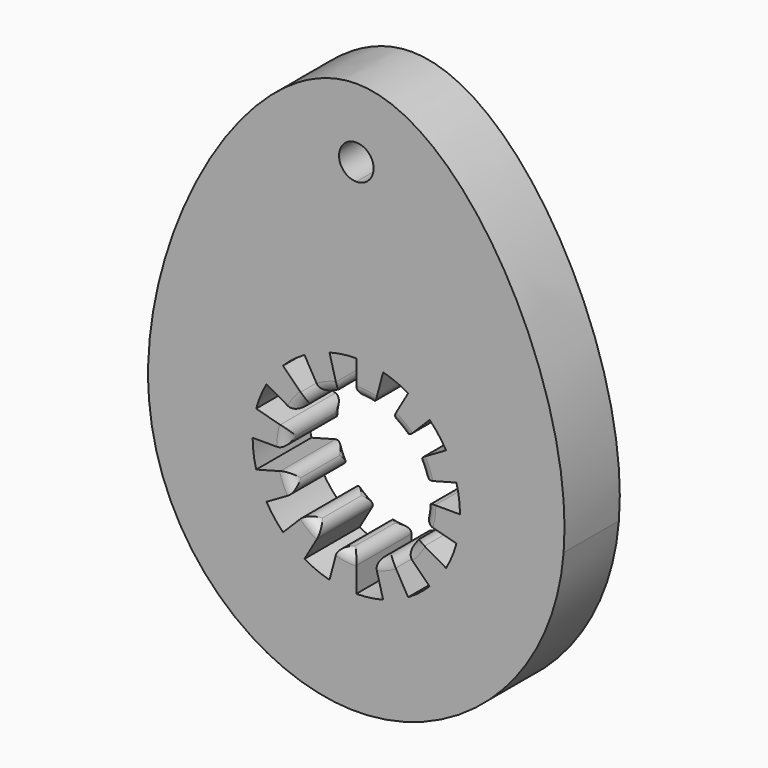
from build123d import *

# Parameters (mm, degrees)
F1_DEPTH = 12.7
F2_R     = 1.905


with BuildPart() as f1:
    # F0 (on Front) → F1 (new body)
    with BuildSketch(Plane.XZ):
        with BuildLine():
            ThreePointArc((18.4008869908, 4.9305028092), (18.8870246092, 2.4865239618), (19.05, 0))
            Line((19.05, 0), (38.1, 0))
            add(Edge.make_bspline(
                [(38.1, 0), (40.2886501107, 26.66795404), (20.1443250553, 63.5), (0, 63.5)],
                knots=[0.7301671149, 0.7301671149, 0.7301671149, 0.7301671149, 1, 1, 1, 1], degree=3))
            Line((0, 63.5), (0, 53.975))
            ThreePointArc((0, 53.975), (2.2450640303, 53.0450640303), (3.175, 50.8))
            ThreePointArc((3.175, 50.8), (2.2450640303, 48.5549359697), (0, 47.625))
            Line((0, 47.625), (0, 19.05))
            ThreePointArc((0, 19.05), (2.4865239618, 18.8870246092), (4.9305028092, 18.4008869908))
            ThreePointArc((4.9305028092, 18.4008869908), (7.2901193866, 17.5999050943), (9.525, 16.4977839421))
            ThreePointArc((9.525, 16.4977839421), (11.5969052226, 15.1133811325), (13.4703841816, 13.4703841816))
            ThreePointArc((13.4703841816, 13.4703841816), (15.1133811325, 11.5969052226), (16.4977839421, 9.525))
            ThreePointArc((16.4977839421, 9.525), (17.5999050943, 7.2901193866), (18.4008869908, 4.9305028092))
        make_face()
        with BuildLine():
            Line((38.1, 0), (19.05, 0))
            ThreePointArc((19.05, 0), (18.8870246092, -2.4865239618), (18.4008869908, -4.9305028092))
            ThreePointArc((18.4008869908, -4.9305028092), (17.5999050943, -7.2901193866), (16.4977839421, -9.525))
            ThreePointArc((16.4977839421, -9.525), (15.1133811325, -11.5969052226), (13.4703841816, -13.4703841816))
            ThreePointArc((13.4703841816, -13.4703841816), (11.5969052226, -15.1133811325), (9.525, -16.4977839421))
            ThreePointArc((9.525, -16.4977839421), (7.2901193866, -17.5999050943), (4.9305028092, -18.4008869908))
            ThreePointArc((4.9305028092, -18.4008869908), (2.4865239618, -18.8870246092), (0, -19.05))
            Line((0, -19.05), (0, -38.1))
            add(Edge.make_bspline(
                [(0, -38.1), (18.1165420908, -38.1), (36.2330841816, -22.7477315801), (38.1, 0)],
                knots=[0.5, 0.5, 0.5, 0.5, 0.7301671149, 0.7301671149, 0.7301671149, 0.7301671149], degree=3))
        make_face()
        with BuildLine():
            ThreePointArc((-18.4008869908, -4.9305028092), (-18.8870246092, -2.4865239618), (-19.05, 0))
            Line((-19.05, 0), (-38.1, 0))
            add(Edge.make_bspline(
                [(-38.1, 0), (-36.2330841816, -22.7477315801), (-18.1165420908, -38.1), (0, -38.1)],
                knots=[0.2698328851, 0.2698328851, 0.2698328851, 0.2698328851, 0.5, 0.5, 0.5, 0.5], degree=3))
            Line((0, -38.1), (0, -19.05))
            ThreePointArc((0, -19.05), (-2.4865239618, -18.8870246092), (-4.9305028092, -18.4008869908))
            ThreePointArc((-4.9305028092, -18.4008869908), (-7.2901193866, -17.5999050943), (-9.525, -16.4977839421))
            ThreePointArc((-9.525, -16.4977839421), (-11.5969052226, -15.1133811325), (-13.4703841816, -13.4703841816))
            ThreePointArc((-13.4703841816, -13.4703841816), (-15.1133811325, -11.5969052226), (-16.4977839421, -9.525))
            ThreePointArc((-16.4977839421, -9.525), (-17.5999050943, -7.2901193866), (-18.4008869908, -4.9305028092))
        make_face()
        with BuildLine():
            Line((-38.1, 0), (-19.05, 0))
            ThreePointArc((-19.05, 0), (-18.8870246092, 2.4865239618), (-18.4008869908, 4.9305028092))
            ThreePointArc((-18.4008869908, 4.9305028092), (-17.5999050943, 7.2901193866), (-16.4977839421, 9.525))
            ThreePointArc((-16.4977839421, 9.525), (-15.1133811325, 11.5969052226), (-13.4703841816, 13.4703841816))
            ThreePointArc((-13.4703841816, 13.4703841816), (-11.5969052226, 15.1133811325), (-9.525, 16.4977839421))
            ThreePointArc((-9.525, 16.4977839421), (-7.2901193866, 17.5999050943), (-4.9305028092, 18.4008869908))
            ThreePointArc((-4.9305028092, 18.4008869908), (-2.4865239618, 18.8870246092), (0, 19.05))
            Line((0, 19.05), (0, 47.625))
            ThreePointArc((0, 47.625), (-3.175, 50.8), (0, 53.975))
            Line((0, 53.975), (0, 63.5))
            add(Edge.make_bspline(
                [(0, 63.5), (-20.1443250553, 63.5), (-40.2886501107, 26.66795404), (-38.1, 0)],
                knots=[0, 0, 0, 0, 0.2698328851, 0.2698328851, 0.2698328851, 0.2698328851], degree=3))
        make_face()
        with BuildLine():
            Line((-19.05, 0), (-12.7, 0))
            ThreePointArc((-12.7, 0), (-12.5913497394, 1.6576826412), (-12.2672579939, 3.2870018728))
            Line((-12.2672579939, 3.2870018728), (-18.4008869908, 4.9305028092))
            ThreePointArc((-18.4008869908, 4.9305028092), (-18.8870246092, 2.4865239618), (-19.05, 0))
        make_face()
        with BuildLine():
            ThreePointArc((-10.9985226281, 6.35), (-10.0755874217, 7.7312701484), (-8.9802561211, 8.9802561211))
            Line((-8.9802561211, 8.9802561211), (-13.4703841816, 13.4703841816))
            ThreePointArc((-13.4703841816, 13.4703841816), (-15.1133811325, 11.5969052226), (-16.4977839421, 9.525))
            Line((-16.4977839421, 9.525), (-10.9985226281, 6.35))
        make_face()
        with BuildLine():
            ThreePointArc((-6.35, 10.9985226281), (-4.860079591, 11.7332700629), (-3.2870018728, 12.2672579939))
            Line((-3.2870018728, 12.2672579939), (-4.9305028092, 18.4008869908))
            ThreePointArc((-4.9305028092, 18.4008869908), (-7.2901193866, 17.5999050943), (-9.525, 16.4977839421))
            Line((-9.525, 16.4977839421), (-6.35, 10.9985226281))
        make_face()
        with BuildLine():
            Line((0, 19.05), (0, 12.7))
            ThreePointArc((0, 12.7), (1.6576826412, 12.5913497394), (3.2870018728, 12.2672579939))
            Line((3.2870018728, 12.2672579939), (4.9305028092, 18.4008869908))
            ThreePointArc((4.9305028092, 18.4008869908), (2.4865239618, 18.8870246092), (0, 19.05))
        make_face()
        with BuildLine():
            Line((9.525, 16.4977839421), (6.35, 10.9985226281))
            ThreePointArc((6.35, 10.9985226281), (7.7312701484, 10.0755874217), (8.9802561211, 8.9802561211))
            Line((8.9802561211, 8.9802561211), (13.4703841816, 13.4703841816))
            ThreePointArc((13.4703841816, 13.4703841816), (11.5969052226, 15.1133811325), (9.525, 16.4977839421))
        make_face()
        with BuildLine():
            Line((16.4977839421, 9.525), (10.9985226281, 6.35))
            ThreePointArc((10.9985226281, 6.35), (11.7332700629, 4.860079591), (12.2672579939, 3.2870018728))
            Line((12.2672579939, 3.2870018728), (18.4008869908, 4.9305028092))
            ThreePointArc((18.4008869908, 4.9305028092), (17.5999050943, 7.2901193866), (16.4977839421, 9.525))
        make_face()
        with BuildLine():
            Line((19.05, 0), (12.7, 0))
            ThreePointArc((12.7, 0), (12.5913497394, -1.6576826412), (12.2672579939, -3.2870018728))
            Line((12.2672579939, -3.2870018728), (18.4008869908, -4.9305028092))
            ThreePointArc((18.4008869908, -4.9305028092), (18.8870246092, -2.4865239618), (19.05, 0))
        make_face()
        with BuildLine():
            Line((16.4977839421, -9.525), (10.9985226281, -6.35))
            ThreePointArc((10.9985226281, -6.35), (10.0755874217, -7.7312701484), (8.9802561211, -8.9802561211))
            Line((8.9802561211, -8.9802561211), (13.4703841816, -13.4703841816))
            ThreePointArc((13.4703841816, -13.4703841816), (15.1133811325, -11.5969052226), (16.4977839421, -9.525))
        make_face()
        with BuildLine():
            Line((9.525, -16.4977839421), (6.35, -10.9985226281))
            ThreePointArc((6.35, -10.9985226281), (4.860079591, -11.7332700629), (3.2870018728, -12.2672579939))
            Line((3.2870018728, -12.2672579939), (4.9305028092, -18.4008869908))
            ThreePointArc((4.9305028092, -18.4008869908), (7.2901193866, -17.5999050943), (9.525, -16.4977839421))
        make_face()
        with BuildLine():
            Line((0, -19.05), (0, -12.7))
            ThreePointArc((0, -12.7), (-1.6576826412, -12.5913497394), (-3.2870018728, -12.2672579939))
            Line((-3.2870018728, -12.2672579939), (-4.9305028092, -18.4008869908))
            ThreePointArc((-4.9305028092, -18.4008869908), (-2.4865239618, -18.8870246092), (0, -19.05))
        make_face()
        with BuildLine():
            Line((-9.525, -16.4977839421), (-6.35, -10.9985226281))
            ThreePointArc((-6.35, -10.9985226281), (-7.7312701484, -10.0755874217), (-8.9802561211, -8.9802561211))
            Line((-8.9802561211, -8.9802561211), (-13.4703841816, -13.4703841816))
            ThreePointArc((-13.4703841816, -13.4703841816), (-11.5969052226, -15.1133811325), (-9.525, -16.4977839421))
        make_face()
        with BuildLine():
            Line((-16.4977839421, -9.525), (-10.9985226281, -6.35))
            ThreePointArc((-10.9985226281, -6.35), (-11.7332700629, -4.860079591), (-12.2672579939, -3.2870018728))
            Line((-12.2672579939, -3.2870018728), (-18.4008869908, -4.9305028092))
            ThreePointArc((-18.4008869908, -4.9305028092), (-17.5999050943, -7.2901193866), (-16.4977839421, -9.525))
        make_face()
    extrude(amount=F1_DEPTH)

    # F2
    f2_edges = [f1.edges().sort_by_distance(p)[0] for p in [
        (10.998523, -6.35, 6.35),
        (12.267258, -6.35, 3.287002),
        (11.73327, 0, 4.86008),
        (11.73327, -12.7, 4.86008),
        (12.7, -6.35, 0),
        (12.267258, -6.35, -3.287002),
        (12.59135, 0, -1.657683),
        (12.59135, -12.7, -1.657683),
        (10.998523, -6.35, -6.35),
        (8.980256, -6.35, -8.980256),
        (10.075587, 0, -7.73127),
        (10.075587, -12.7, -7.73127),
        (0, -6.35, 12.7),
        (3.287002, -6.35, 12.267258),
        (1.657683, 0, 12.59135),
        (1.657683, -12.7, 12.59135),
        (6.35, -6.35, 10.998523),
        (8.980256, -6.35, 8.980256),
        (7.73127, 0, 10.075587),
        (7.73127, -12.7, 10.075587),
        (-6.35, -6.35, 10.998523),
        (-3.287002, -6.35, 12.267258),
        (-4.86008, 0, 11.73327),
        (-4.86008, -12.7, 11.73327),
        (-10.998523, -6.35, 6.35),
        (-8.980256, -6.35, 8.980256),
        (-10.075587, 0, 7.73127),
        (-10.075587, -12.7, 7.73127),
        (-12.7, -6.35, 0),
        (-12.267258, -6.35, 3.287002),
        (-12.59135, 0, 1.657683),
        (-12.59135, -12.7, 1.657683),
        (-10.998523, -6.35, -6.35),
        (-12.267258, -6.35, -3.287002),
        (-11.73327, 0, -4.86008),
        (-11.73327, -12.7, -4.86008),
        (-6.35, -6.35, -10.998523),
        (-8.980256, -6.35, -8.980256),
        (-7.73127, 0, -10.075587),
        (-7.73127, -12.7, -10.075587),
        (0, -6.35, -12.7),
        (-3.287002, -6.35, -12.267258),
        (-1.657683, 0, -12.59135),
        (-1.657683, -12.7, -12.59135),
        (6.35, -6.35, -10.998523),
        (3.287002, -6.35, -12.267258),
        (4.86008, 0, -11.73327),
        (4.86008, -12.7, -11.73327),
    ]]
    fillet(f2_edges, radius=F2_R)


solid = f1.part
